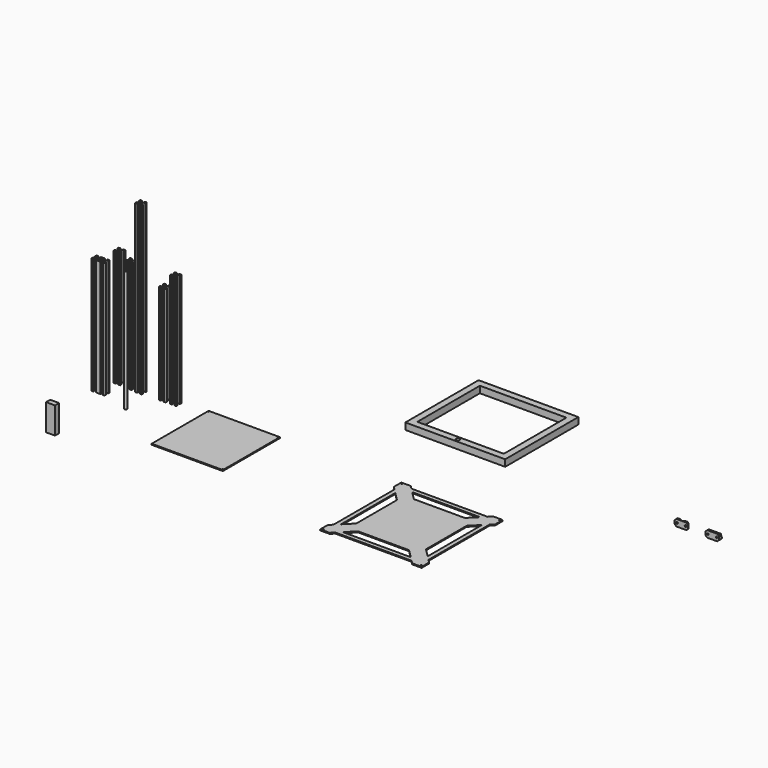
from build123d import *

# Parameters (mm, degrees)
F3_R         = 2.1
F4_DEPTH     = 350
F2_R         = 2.1
F5_DEPTH     = 500
F6_W         = 214
F6_H         = 214
F6_R         = 1.5
F7_DEPTH     = 3
F0_R         = 2.1
F8_DEPTH     = 350
F9_R         = 2
F10_DEPTH    = 3
F1_R         = 2.1
F11_DEPTH    = 335
F12_R        = 4
F13_DEPTH    = 365
F14_W        = 26.9409120083
F14_H        = 15.4066830873
F15_DEPTH    = 80
F16_R        = 2.1
F17_DEPTH    = 300
F18_R        = 2.1
F19_DEPTH    = 340
F20_R        = 5.6486540252
F20_W        = 260
F20_H        = 20
F21_DEPTH    = 20
F22_W        = 40
F22_H        = 15
F22_R        = 2
F23_DEPTH    = 20
F24_R        = 6
F25_DEPTH    = 10
F26_R        = 2.75
F27_DEPTH    = 25
F28_T1_DEPTH = 86.8637576871
F29_W        = 40
F29_H        = 23.6347752469
F29_R        = 2
F30_DEPTH    = 20
F31_R        = 6
F32_DEPTH    = 18
F33_R        = 2.25
F34_DEPTH    = 25
F35_T1_DEPTH = 81.7203917112
F36_W        = 47.229886055
F36_H        = 17.0893235207
F37_DEPTH    = 18
F38_SIZE     = 5
F39_W        = 52.9752969742
F39_H        = 17.0372793525
F40_DEPTH    = 10
F41_R        = 7.6141041327
F42_DEPTH    = 12
F43_SIZE     = 5
F44_SIZE     = 2


# Not quite as in the source:
# - a fillet or chamfer that OpenCascade refuses, or shapes differently, is made with other operations: its cross-section is extruded or revolved along the edge and cut away or added


with BuildPart() as f4:
    # F3 (on Top) → F4 (new body)
    with BuildSketch(Plane.XY):
        with BuildLine():
            Line((-71.2157925161, -12.9482020284), (-74.8085638019, -12.9482020284))
            ThreePointArc((-74.8085638019, -12.9482020284), (-75.8692239736, -13.3875418566), (-76.3085638019, -14.4482020284))
            Line((-76.3085638019, -14.4482020284), (-76.3085638019, -18.0409733141))
            ThreePointArc((-76.3085638019, -18.0409733141), (-76.2484286325, -18.3432932257), (-76.077178159, -18.5995876712))
            Line((-76.077178159, -18.5995876712), (-74.6185638019, -20.0582020284))
            Line((-74.6185638019, -20.0582020284), (-74.5085638019, -20.0582020284))
            Line((-74.5085638019, -20.0582020284), (-74.5085638019, -17.4482020284))
            Line((-74.5085638019, -17.4482020284), (-72.8692239736, -17.4482020284))
            Line((-72.8692239736, -17.4482020284), (-69.7085638019, -20.6088622002))
            Line((-69.7085638019, -20.6088622002), (-69.7085638019, -25.2875418566))
            Line((-69.7085638019, -25.2875418566), (-72.8692239736, -28.4482020284))
            Line((-72.8692239736, -28.4482020284), (-74.5085638019, -28.4482020284))
            Line((-74.5085638019, -28.4482020284), (-74.5085638019, -25.8382020284))
            Line((-74.5085638019, -25.8382020284), (-74.6185638019, -25.8382020284))
            Line((-74.6185638019, -25.8382020284), (-76.077178159, -27.2968163855))
            ThreePointArc((-76.077178159, -27.2968163855), (-76.2484286325, -27.5531108311), (-76.3085638019, -27.8554307427))
            Line((-76.3085638019, -27.8554307427), (-76.3085638019, -31.4482020284))
            ThreePointArc((-76.3085638019, -31.4482020284), (-75.8692239736, -32.5088622002), (-74.8085638019, -32.9482020284))
            Line((-74.8085638019, -32.9482020284), (-71.2157925161, -32.9482020284))
            ThreePointArc((-71.2157925161, -32.9482020284), (-70.9134726046, -32.8880668591), (-70.657178159, -32.7168163855))
            Line((-70.657178159, -32.7168163855), (-69.1985638019, -31.2582020284))
            Line((-69.1985638019, -31.2582020284), (-69.1985638019, -31.1482020284))
            Line((-69.1985638019, -31.1482020284), (-71.8085638019, -31.1482020284))
            Line((-71.8085638019, -31.1482020284), (-71.8085638019, -29.5088622002))
            Line((-71.8085638019, -29.5088622002), (-68.6479036301, -26.3482020284))
            Line((-68.6479036301, -26.3482020284), (-63.9692239736, -26.3482020284))
            Line((-63.9692239736, -26.3482020284), (-60.8085638019, -29.5088622002))
            Line((-60.8085638019, -29.5088622002), (-60.8085638019, -31.1482020284))
            Line((-60.8085638019, -31.1482020284), (-63.4185638019, -31.1482020284))
            Line((-63.4185638019, -31.1482020284), (-63.4185638019, -31.2582020284))
            Line((-63.4185638019, -31.2582020284), (-61.9599494447, -32.7168163855))
            ThreePointArc((-61.9599494447, -32.7168163855), (-61.7036549992, -32.8880668591), (-61.4013350876, -32.9482020284))
            Line((-61.4013350876, -32.9482020284), (-57.8085638019, -32.9482020284))
            Line((-57.8085638019, -32.9482020284), (-54.8085638019, -32.9482020284))
            Line((-54.8085638019, -32.9482020284), (-51.2157925161, -32.9482020284))
            ThreePointArc((-51.2157925161, -32.9482020284), (-50.9134726046, -32.8880668591), (-50.657178159, -32.7168163855))
            Line((-50.657178159, -32.7168163855), (-49.1985638019, -31.2582020284))
            Line((-49.1985638019, -31.2582020284), (-49.1985638019, -31.1482020284))
            Line((-49.1985638019, -31.1482020284), (-51.8085638019, -31.1482020284))
            Line((-51.8085638019, -31.1482020284), (-51.8085638019, -29.5088622002))
            Line((-51.8085638019, -29.5088622002), (-48.6479036301, -26.3482020284))
            Line((-48.6479036301, -26.3482020284), (-43.9692239736, -26.3482020284))
            Line((-43.9692239736, -26.3482020284), (-40.8085638019, -29.5088622002))
            Line((-40.8085638019, -29.5088622002), (-40.8085638019, -31.1482020284))
            Line((-40.8085638019, -31.1482020284), (-43.4185638019, -31.1482020284))
            Line((-43.4185638019, -31.1482020284), (-43.4185638019, -31.2582020284))
            Line((-43.4185638019, -31.2582020284), (-41.9599494447, -32.7168163855))
            ThreePointArc((-41.9599494447, -32.7168163855), (-41.7036549992, -32.8880668591), (-41.4013350876, -32.9482020284))
            Line((-41.4013350876, -32.9482020284), (-37.8085638019, -32.9482020284))
            ThreePointArc((-37.8085638019, -32.9482020284), (-36.7479036301, -32.5088622002), (-36.3085638019, -31.4482020284))
            Line((-36.3085638019, -31.4482020284), (-36.3085638019, -27.8554307427))
            ThreePointArc((-36.3085638019, -27.8554307427), (-36.3686989712, -27.5531108311), (-36.5399494447, -27.2968163855))
            Line((-36.5399494447, -27.2968163855), (-37.9985638019, -25.8382020284))
            Line((-37.9985638019, -25.8382020284), (-38.1085638019, -25.8382020284))
            Line((-38.1085638019, -25.8382020284), (-38.1085638019, -28.4482020284))
            Line((-38.1085638019, -28.4482020284), (-39.7479036301, -28.4482020284))
            Line((-39.7479036301, -28.4482020284), (-42.9085638019, -25.2875418566))
            Line((-42.9085638019, -25.2875418566), (-42.9085638019, -20.6088622002))
            Line((-42.9085638019, -20.6088622002), (-39.7479036301, -17.4482020284))
            Line((-39.7479036301, -17.4482020284), (-38.1085638019, -17.4482020284))
            Line((-38.1085638019, -17.4482020284), (-38.1085638019, -20.0582020284))
            Line((-38.1085638019, -20.0582020284), (-37.9985638019, -20.0582020284))
            Line((-37.9985638019, -20.0582020284), (-36.5399494447, -18.5995876712))
            ThreePointArc((-36.5399494447, -18.5995876712), (-36.3686989712, -18.3432932257), (-36.3085638019, -18.0409733141))
            Line((-36.3085638019, -18.0409733141), (-36.3085638019, -14.4482020284))
            ThreePointArc((-36.3085638019, -14.4482020284), (-36.7479036301, -13.3875418566), (-37.8085638019, -12.9482020284))
            Line((-37.8085638019, -12.9482020284), (-41.4013350876, -12.9482020284))
            ThreePointArc((-41.4013350876, -12.9482020284), (-41.7036549992, -13.0083371977), (-41.9599494447, -13.1795876712))
            Line((-41.9599494447, -13.1795876712), (-43.4185638019, -14.6382020284))
            Line((-43.4185638019, -14.6382020284), (-43.4185638019, -14.7482020284))
            Line((-43.4185638019, -14.7482020284), (-40.8085638019, -14.7482020284))
            Line((-40.8085638019, -14.7482020284), (-40.8085638019, -16.3875418566))
            Line((-40.8085638019, -16.3875418566), (-43.9692239736, -19.5482020284))
            Line((-43.9692239736, -19.5482020284), (-48.6479036301, -19.5482020284))
            Line((-48.6479036301, -19.5482020284), (-51.8085638019, -16.3875418566))
            Line((-51.8085638019, -16.3875418566), (-51.8085638019, -14.7482020284))
            Line((-51.8085638019, -14.7482020284), (-49.1985638019, -14.7482020284))
            Line((-49.1985638019, -14.7482020284), (-49.1985638019, -14.6382020284))
            Line((-49.1985638019, -14.6382020284), (-50.657178159, -13.1795876712))
            ThreePointArc((-50.657178159, -13.1795876712), (-50.9134726046, -13.0083371977), (-51.2157925161, -12.9482020284))
            Line((-51.2157925161, -12.9482020284), (-54.8085638019, -12.9482020284))
            Line((-54.8085638019, -12.9482020284), (-57.8085638019, -12.9482020284))
            Line((-57.8085638019, -12.9482020284), (-61.4013350876, -12.9482020284))
            ThreePointArc((-61.4013350876, -12.9482020284), (-61.7036549992, -13.0083371977), (-61.9599494447, -13.1795876712))
            Line((-61.9599494447, -13.1795876712), (-63.4185638019, -14.6382020284))
            Line((-63.4185638019, -14.6382020284), (-63.4185638019, -14.7482020284))
            Line((-63.4185638019, -14.7482020284), (-60.8085638019, -14.7482020284))
            Line((-60.8085638019, -14.7482020284), (-60.8085638019, -16.3875418566))
            Line((-60.8085638019, -16.3875418566), (-63.9692239736, -19.5482020284))
            Line((-63.9692239736, -19.5482020284), (-68.6479036301, -19.5482020284))
            Line((-68.6479036301, -19.5482020284), (-71.8085638019, -16.3875418566))
            Line((-71.8085638019, -16.3875418566), (-71.8085638019, -14.7482020284))
            Line((-71.8085638019, -14.7482020284), (-69.1985638019, -14.7482020284))
            Line((-69.1985638019, -14.7482020284), (-69.1985638019, -14.6382020284))
            Line((-69.1985638019, -14.6382020284), (-70.657178159, -13.1795876712))
            ThreePointArc((-70.657178159, -13.1795876712), (-70.9134726046, -13.0083371977), (-71.2157925161, -12.9482020284))
        make_face()
        Polygon((-74.5085638019, -29.5182020284), (-73.9685638019, -29.5182020284), (-72.8785638019, -30.6082020284), (-72.8785638019, -31.1482020284), (-74.5085638019, -31.1482020284), align=None, mode=Mode.SUBTRACT)
        Polygon((-58.6485638019, -29.5182020284), (-58.1085638019, -29.5182020284), (-58.1085638019, -31.1482020284), (-59.7385638019, -31.1482020284), (-59.7385638019, -30.6082020284), align=None, mode=Mode.SUBTRACT)
        Polygon((-54.5085638019, -31.1482020284), (-54.5085638019, -29.5182020284), (-53.9685638019, -29.5182020284), (-52.8785638019, -30.6082020284), (-52.8785638019, -31.1482020284), align=None, mode=Mode.SUBTRACT)
        Polygon((-39.7385638019, -30.6082020284), (-38.6485638019, -29.5182020284), (-38.1085638019, -29.5182020284), (-38.1085638019, -31.1482020284), (-39.7385638019, -31.1482020284), align=None, mode=Mode.SUBTRACT)
        with BuildLine():
            Line((-59.7479036301, -28.4482020284), (-62.9085638019, -25.2875418566))
            Line((-62.9085638019, -25.2875418566), (-62.9085638019, -23.6909259111))
            Line((-62.9085638019, -23.6909259111), (-58.2713541983, -23.6909259111))
            ThreePointArc((-58.2713541983, -23.6909259111), (-56.3085638019, -25.0468170256), (-54.3457734054, -23.6909259111))
            Line((-54.3457734054, -23.6909259111), (-49.7085638019, -23.6909259111))
            Line((-49.7085638019, -23.6909259111), (-49.7085638019, -25.2875418566))
            Line((-49.7085638019, -25.2875418566), (-52.8692239736, -28.4482020284))
            Line((-52.8692239736, -28.4482020284), (-54.5085638019, -28.4482020284))
            Line((-54.5085638019, -28.4482020284), (-58.1085638019, -28.4482020284))
            Line((-58.1085638019, -28.4482020284), (-59.7479036301, -28.4482020284))
        make_face(mode=Mode.SUBTRACT)
        with Locations((-66.3085638019, -22.9482020284)):
            Circle(F3_R, mode=Mode.SUBTRACT)
        Polygon((-74.5085638019, -14.7482020284), (-72.8785638019, -14.7482020284), (-72.8785638019, -15.2882020284), (-73.9685638019, -16.3782020284), (-74.5085638019, -16.3782020284), align=None, mode=Mode.SUBTRACT)
        Polygon((-58.1085638019, -14.7482020284), (-58.1085638019, -16.3782020284), (-58.6485638019, -16.3782020284), (-59.7385638019, -15.2882020284), (-59.7385638019, -14.7482020284), align=None, mode=Mode.SUBTRACT)
        with BuildLine():
            Line((-62.9085638019, -22.2054781457), (-62.9085638019, -20.6088622002))
            Line((-62.9085638019, -20.6088622002), (-59.7479036301, -17.4482020284))
            Line((-59.7479036301, -17.4482020284), (-58.1085638019, -17.4482020284))
            Line((-58.1085638019, -17.4482020284), (-54.5085638019, -17.4482020284))
            Line((-54.5085638019, -17.4482020284), (-52.8692239736, -17.4482020284))
            Line((-52.8692239736, -17.4482020284), (-49.7085638019, -20.6088622002))
            Line((-49.7085638019, -20.6088622002), (-49.7085638019, -22.2054781457))
            Line((-49.7085638019, -22.2054781457), (-54.3457734054, -22.2054781457))
            ThreePointArc((-54.3457734054, -22.2054781457), (-56.3085638019, -20.8495870312), (-58.2713541983, -22.2054781457))
            Line((-58.2713541983, -22.2054781457), (-62.9085638019, -22.2054781457))
        make_face(mode=Mode.SUBTRACT)
        with Locations((-46.3085638019, -22.9482020284)):
            Circle(F3_R, mode=Mode.SUBTRACT)
        Polygon((-52.8785638019, -15.2882020284), (-53.9685638019, -16.3782020284), (-54.5085638019, -16.3782020284), (-54.5085638019, -14.7482020284), (-52.8785638019, -14.7482020284), align=None, mode=Mode.SUBTRACT)
        Polygon((-38.6485638019, -16.3782020284), (-39.7385638019, -15.2882020284), (-39.7385638019, -14.7482020284), (-38.1085638019, -14.7482020284), (-38.1085638019, -16.3782020284), align=None, mode=Mode.SUBTRACT)
    extrude(amount=F4_DEPTH)


with BuildPart() as f5:
    # F2 (on Top) → F5 (new body)
    with BuildSketch(Plane.XY):
        with BuildLine():
            Line((12.9063250926, 46.0312701171), (9.3135538069, 46.0312701171))
            ThreePointArc((9.3135538069, 46.0312701171), (8.2528936351, 45.5919302888), (7.8135538069, 44.5312701171))
            Line((7.8135538069, 44.5312701171), (7.8135538069, 40.9384988313))
            ThreePointArc((7.8135538069, 40.9384988313), (7.8736889762, 40.6361789198), (8.0449394498, 40.3798844742))
            Line((8.0449394498, 40.3798844742), (9.5035538069, 38.9212701171))
            Line((9.5035538069, 38.9212701171), (9.6135538069, 38.9212701171))
            Line((9.6135538069, 38.9212701171), (9.6135538069, 41.5312701171))
            Line((9.6135538069, 41.5312701171), (11.2528936351, 41.5312701171))
            Line((11.2528936351, 41.5312701171), (14.4135538069, 38.3706099453))
            Line((14.4135538069, 38.3706099453), (14.4135538069, 33.6919302888))
            Line((14.4135538069, 33.6919302888), (11.2528936351, 30.5312701171))
            Line((11.2528936351, 30.5312701171), (9.6135538069, 30.5312701171))
            Line((9.6135538069, 30.5312701171), (9.6135538069, 33.1412701171))
            Line((9.6135538069, 33.1412701171), (9.5035538069, 33.1412701171))
            Line((9.5035538069, 33.1412701171), (8.0449394498, 31.6826557599))
            ThreePointArc((8.0449394498, 31.6826557599), (7.8736889762, 31.4263613144), (7.8135538069, 31.1240414028))
            Line((7.8135538069, 31.1240414028), (7.8135538069, 27.5312701171))
            ThreePointArc((7.8135538069, 27.5312701171), (8.2528936351, 26.4706099453), (9.3135538069, 26.0312701171))
            Line((9.3135538069, 26.0312701171), (12.9063250926, 26.0312701171))
            ThreePointArc((12.9063250926, 26.0312701171), (13.2086450042, 26.0914052864), (13.4649394498, 26.2626557599))
            Line((13.4649394498, 26.2626557599), (14.9235538069, 27.7212701171))
            Line((14.9235538069, 27.7212701171), (14.9235538069, 27.8312701171))
            Line((14.9235538069, 27.8312701171), (12.3135538069, 27.8312701171))
            Line((12.3135538069, 27.8312701171), (12.3135538069, 29.4706099453))
            Line((12.3135538069, 29.4706099453), (15.4742139787, 32.6312701171))
            Line((15.4742139787, 32.6312701171), (20.1528936351, 32.6312701171))
            Line((20.1528936351, 32.6312701171), (23.3135538069, 29.4706099453))
            Line((23.3135538069, 29.4706099453), (23.3135538069, 27.8312701171))
            Line((23.3135538069, 27.8312701171), (20.7035538069, 27.8312701171))
            Line((20.7035538069, 27.8312701171), (20.7035538069, 27.7212701171))
            Line((20.7035538069, 27.7212701171), (22.1621681641, 26.2626557599))
            ThreePointArc((22.1621681641, 26.2626557599), (22.4184626096, 26.0914052864), (22.7207825212, 26.0312701171))
            Line((22.7207825212, 26.0312701171), (26.3135538069, 26.0312701171))
            ThreePointArc((26.3135538069, 26.0312701171), (27.3742139787, 26.4706099453), (27.8135538069, 27.5312701171))
            Line((27.8135538069, 27.5312701171), (27.8135538069, 31.1240414028))
            ThreePointArc((27.8135538069, 31.1240414028), (27.7534186376, 31.4263613144), (27.5821681641, 31.6826557599))
            Line((27.5821681641, 31.6826557599), (26.1235538069, 33.1412701171))
            Line((26.1235538069, 33.1412701171), (26.0135538069, 33.1412701171))
            Line((26.0135538069, 33.1412701171), (26.0135538069, 30.5312701171))
            Line((26.0135538069, 30.5312701171), (24.3742139787, 30.5312701171))
            Line((24.3742139787, 30.5312701171), (21.2135538069, 33.6919302888))
            Line((21.2135538069, 33.6919302888), (21.2135538069, 38.3706099453))
            Line((21.2135538069, 38.3706099453), (24.3742139787, 41.5312701171))
            Line((24.3742139787, 41.5312701171), (26.0135538069, 41.5312701171))
            Line((26.0135538069, 41.5312701171), (26.0135538069, 38.9212701171))
            Line((26.0135538069, 38.9212701171), (26.1235538069, 38.9212701171))
            Line((26.1235538069, 38.9212701171), (27.5821681641, 40.3798844742))
            ThreePointArc((27.5821681641, 40.3798844742), (27.7534186376, 40.6361789198), (27.8135538069, 40.9384988313))
            Line((27.8135538069, 40.9384988313), (27.8135538069, 44.5312701171))
            ThreePointArc((27.8135538069, 44.5312701171), (27.3742139787, 45.5919302888), (26.3135538069, 46.0312701171))
            Line((26.3135538069, 46.0312701171), (22.7207825212, 46.0312701171))
            ThreePointArc((22.7207825212, 46.0312701171), (22.4184626096, 45.9711349477), (22.1621681641, 45.7998844742))
            Line((22.1621681641, 45.7998844742), (20.7035538069, 44.3412701171))
            Line((20.7035538069, 44.3412701171), (20.7035538069, 44.2312701171))
            Line((20.7035538069, 44.2312701171), (23.3135538069, 44.2312701171))
            Line((23.3135538069, 44.2312701171), (23.3135538069, 42.5919302888))
            Line((23.3135538069, 42.5919302888), (20.1528936351, 39.4312701171))
            Line((20.1528936351, 39.4312701171), (15.4742139787, 39.4312701171))
            Line((15.4742139787, 39.4312701171), (12.3135538069, 42.5919302888))
            Line((12.3135538069, 42.5919302888), (12.3135538069, 44.2312701171))
            Line((12.3135538069, 44.2312701171), (14.9235538069, 44.2312701171))
            Line((14.9235538069, 44.2312701171), (14.9235538069, 44.3412701171))
            Line((14.9235538069, 44.3412701171), (13.4649394498, 45.7998844742))
            ThreePointArc((13.4649394498, 45.7998844742), (13.2086450042, 45.9711349477), (12.9063250926, 46.0312701171))
        make_face()
        Polygon((9.6135538069, 29.4612701171), (10.1535538069, 29.4612701171), (11.2435538069, 28.3712701171), (11.2435538069, 27.8312701171), (9.6135538069, 27.8312701171), align=None, mode=Mode.SUBTRACT)
        Polygon((25.4735538069, 29.4612701171), (26.0135538069, 29.4612701171), (26.0135538069, 27.8312701171), (24.3835538069, 27.8312701171), (24.3835538069, 28.3712701171), align=None, mode=Mode.SUBTRACT)
        with Locations((17.8135538069, 36.0312701171)):
            Circle(F2_R, mode=Mode.SUBTRACT)
        Polygon((9.6135538069, 44.2312701171), (11.2435538069, 44.2312701171), (11.2435538069, 43.6912701171), (10.1535538069, 42.6012701171), (9.6135538069, 42.6012701171), align=None, mode=Mode.SUBTRACT)
        Polygon((26.0135538069, 44.2312701171), (26.0135538069, 42.6012701171), (25.4735538069, 42.6012701171), (24.3835538069, 43.6912701171), (24.3835538069, 44.2312701171), align=None, mode=Mode.SUBTRACT)
    extrude(amount=F5_DEPTH)


with BuildPart() as f7:
    # F6 (on Top) → F7 (new body)
    with BuildSketch(Plane.XY):
        with Locations((313.2716193795, -52.2007276407)):
            Rectangle(F6_W, F6_H)
        with Locations((208.7716193795, -156.7007276407)):
            Circle(F6_R, mode=Mode.SUBTRACT)
        with Locations((417.7716193795, -156.7007276407)):
            Circle(F6_R, mode=Mode.SUBTRACT)
        with Locations((208.7716193795, 52.2992723593)):
            Circle(F6_R, mode=Mode.SUBTRACT)
        with Locations((417.7716193795, 52.2992723593)):
            Circle(F6_R, mode=Mode.SUBTRACT)
    extrude(amount=F7_DEPTH)


with BuildPart() as f8:
    # F0 (on Top) → F8 (new body)
    with BuildSketch(Plane.XY):
        with BuildLine():
            Line((-55.2372885438, 50.4958480005), (-58.8300598296, 50.4958480005))
            ThreePointArc((-58.8300598296, 50.4958480005), (-59.8907200014, 50.0565081723), (-60.3300598296, 48.9958480005))
            Line((-60.3300598296, 48.9958480005), (-60.3300598296, 45.4030767148))
            ThreePointArc((-60.3300598296, 45.4030767148), (-60.2699246603, 45.1007568032), (-60.0986741867, 44.8444623577))
            Line((-60.0986741867, 44.8444623577), (-58.6400598296, 43.3858480005))
            Line((-58.6400598296, 43.3858480005), (-58.5300598296, 43.3858480005))
            Line((-58.5300598296, 43.3858480005), (-58.5300598296, 45.9958480005))
            Line((-58.5300598296, 45.9958480005), (-56.8907200014, 45.9958480005))
            Line((-56.8907200014, 45.9958480005), (-53.7300598296, 42.8351878288))
            Line((-53.7300598296, 42.8351878288), (-53.7300598296, 38.1565081723))
            Line((-53.7300598296, 38.1565081723), (-56.8907200014, 34.9958480005))
            Line((-56.8907200014, 34.9958480005), (-58.5300598296, 34.9958480005))
            Line((-58.5300598296, 34.9958480005), (-58.5300598296, 37.6058480005))
            Line((-58.5300598296, 37.6058480005), (-58.6400598296, 37.6058480005))
            Line((-58.6400598296, 37.6058480005), (-60.0986741867, 36.1472336434))
            ThreePointArc((-60.0986741867, 36.1472336434), (-60.2699246603, 35.8909391978), (-60.3300598296, 35.5886192863))
            Line((-60.3300598296, 35.5886192863), (-60.3300598296, 31.9958480005))
            ThreePointArc((-60.3300598296, 31.9958480005), (-59.8907200014, 30.9351878288), (-58.8300598296, 30.4958480005))
            Line((-58.8300598296, 30.4958480005), (-55.2372885438, 30.4958480005))
            ThreePointArc((-55.2372885438, 30.4958480005), (-54.9349686323, 30.5559831699), (-54.6786741867, 30.7272336434))
            Line((-54.6786741867, 30.7272336434), (-53.2200598296, 32.1858480005))
            Line((-53.2200598296, 32.1858480005), (-53.2200598296, 32.2958480005))
            Line((-53.2200598296, 32.2958480005), (-55.8300598296, 32.2958480005))
            Line((-55.8300598296, 32.2958480005), (-55.8300598296, 33.9351878288))
            Line((-55.8300598296, 33.9351878288), (-52.6693996578, 37.0958480005))
            Line((-52.6693996578, 37.0958480005), (-47.9907200014, 37.0958480005))
            Line((-47.9907200014, 37.0958480005), (-44.8300598296, 33.9351878288))
            Line((-44.8300598296, 33.9351878288), (-44.8300598296, 32.2958480005))
            Line((-44.8300598296, 32.2958480005), (-47.4400598296, 32.2958480005))
            Line((-47.4400598296, 32.2958480005), (-47.4400598296, 32.1858480005))
            Line((-47.4400598296, 32.1858480005), (-45.9814454724, 30.7272336434))
            ThreePointArc((-45.9814454724, 30.7272336434), (-45.7251510269, 30.5559831699), (-45.4228311153, 30.4958480005))
            Line((-45.4228311153, 30.4958480005), (-41.8300598296, 30.4958480005))
            ThreePointArc((-41.8300598296, 30.4958480005), (-40.7693996578, 30.9351878288), (-40.3300598296, 31.9958480005))
            Line((-40.3300598296, 31.9958480005), (-40.3300598296, 35.5886192863))
            ThreePointArc((-40.3300598296, 35.5886192863), (-40.3901949989, 35.8909391978), (-40.5614454724, 36.1472336434))
            Line((-40.5614454724, 36.1472336434), (-42.0200598296, 37.6058480005))
            Line((-42.0200598296, 37.6058480005), (-42.1300598296, 37.6058480005))
            Line((-42.1300598296, 37.6058480005), (-42.1300598296, 34.9958480005))
            Line((-42.1300598296, 34.9958480005), (-43.7693996578, 34.9958480005))
            Line((-43.7693996578, 34.9958480005), (-46.9300598296, 38.1565081723))
            Line((-46.9300598296, 38.1565081723), (-46.9300598296, 42.8351878288))
            Line((-46.9300598296, 42.8351878288), (-43.7693996578, 45.9958480005))
            Line((-43.7693996578, 45.9958480005), (-42.1300598296, 45.9958480005))
            Line((-42.1300598296, 45.9958480005), (-42.1300598296, 43.3858480005))
            Line((-42.1300598296, 43.3858480005), (-42.0200598296, 43.3858480005))
            Line((-42.0200598296, 43.3858480005), (-40.5614454724, 44.8444623577))
            ThreePointArc((-40.5614454724, 44.8444623577), (-40.3901949989, 45.1007568032), (-40.3300598296, 45.4030767148))
            Line((-40.3300598296, 45.4030767148), (-40.3300598296, 48.9958480005))
            ThreePointArc((-40.3300598296, 48.9958480005), (-40.7693996578, 50.0565081723), (-41.8300598296, 50.4958480005))
            Line((-41.8300598296, 50.4958480005), (-45.4228311153, 50.4958480005))
            ThreePointArc((-45.4228311153, 50.4958480005), (-45.7251510269, 50.4357128312), (-45.9814454724, 50.2644623577))
            Line((-45.9814454724, 50.2644623577), (-47.4400598296, 48.8058480005))
            Line((-47.4400598296, 48.8058480005), (-47.4400598296, 48.6958480005))
            Line((-47.4400598296, 48.6958480005), (-44.8300598296, 48.6958480005))
            Line((-44.8300598296, 48.6958480005), (-44.8300598296, 47.0565081723))
            Line((-44.8300598296, 47.0565081723), (-47.9907200014, 43.8958480005))
            Line((-47.9907200014, 43.8958480005), (-52.6693996578, 43.8958480005))
            Line((-52.6693996578, 43.8958480005), (-55.8300598296, 47.0565081723))
            Line((-55.8300598296, 47.0565081723), (-55.8300598296, 48.6958480005))
            Line((-55.8300598296, 48.6958480005), (-53.2200598296, 48.6958480005))
            Line((-53.2200598296, 48.6958480005), (-53.2200598296, 48.8058480005))
            Line((-53.2200598296, 48.8058480005), (-54.6786741867, 50.2644623577))
            ThreePointArc((-54.6786741867, 50.2644623577), (-54.9349686323, 50.4357128312), (-55.2372885438, 50.4958480005))
        make_face()
        Polygon((-58.5300598296, 33.9258480005), (-57.9900598296, 33.9258480005), (-56.9000598296, 32.8358480005), (-56.9000598296, 32.2958480005), (-58.5300598296, 32.2958480005), align=None, mode=Mode.SUBTRACT)
        Polygon((-42.6700598296, 33.9258480005), (-42.1300598296, 33.9258480005), (-42.1300598296, 32.2958480005), (-43.7600598296, 32.2958480005), (-43.7600598296, 32.8358480005), align=None, mode=Mode.SUBTRACT)
        with Locations((-50.3300598296, 40.4958480005)):
            Circle(F0_R, mode=Mode.SUBTRACT)
        Polygon((-58.5300598296, 48.6958480005), (-56.9000598296, 48.6958480005), (-56.9000598296, 48.1558480005), (-57.9900598296, 47.0658480005), (-58.5300598296, 47.0658480005), align=None, mode=Mode.SUBTRACT)
        Polygon((-42.1300598296, 48.6958480005), (-42.1300598296, 47.0658480005), (-42.6700598296, 47.0658480005), (-43.7600598296, 48.1558480005), (-43.7600598296, 48.6958480005), align=None, mode=Mode.SUBTRACT)
        with BuildLine():
            ThreePointArc((-60.3300598296, 48.9958480005), (-59.8907200014, 50.0565081723), (-58.8300598296, 50.4958480005))
            Line((-58.8300598296, 50.4958480005), (-60.3300598296, 50.4958480005))
            Line((-60.3300598296, 50.4958480005), (-60.3300598296, 48.9958480005))
        make_face()
        with BuildLine():
            Line((-40.3300598296, 50.4958480005), (-41.8300598296, 50.4958480005))
            ThreePointArc((-41.8300598296, 50.4958480005), (-40.7693996578, 50.0565081723), (-40.3300598296, 48.9958480005))
            Line((-40.3300598296, 48.9958480005), (-40.3300598296, 50.4958480005))
        make_face()
        with BuildLine():
            ThreePointArc((-58.8300598296, 30.4958480005), (-59.8907200014, 30.9351878288), (-60.3300598296, 31.9958480005))
            Line((-60.3300598296, 31.9958480005), (-60.3300598296, 30.4958480005))
            Line((-60.3300598296, 30.4958480005), (-58.8300598296, 30.4958480005))
        make_face()
        with BuildLine():
            Line((-40.3300598296, 30.4958480005), (-40.3300598296, 31.9958480005))
            ThreePointArc((-40.3300598296, 31.9958480005), (-40.7693996578, 30.9351878288), (-41.8300598296, 30.4958480005))
            Line((-41.8300598296, 30.4958480005), (-40.3300598296, 30.4958480005))
        make_face()
    extrude(amount=F8_DEPTH)


with BuildPart() as f10:
    # F9 (on Top) → F10 (new body)
    with BuildSketch(Plane.XY):
        with BuildLine():
            Line((815.4132323337, 52.85364175), (792.1289610863, 52.85364175))
            ThreePointArc((792.1289610863, 52.85364175), (788.5934271803, 51.3891756559), (787.1289610863, 47.85364175))
            Line((787.1289610863, 47.85364175), (787.1289610863, 24.5693705025))
            Line((787.1289610863, 24.5693705025), (796.6539610863, 15.0443705025))
            Line((796.6539610863, 15.0443705025), (796.6539610863, 43.32864175))
            Line((796.6539610863, 43.32864175), (824.9382323337, 43.32864175))
            Line((824.9382323337, 43.32864175), (815.4132323337, 52.85364175))
        make_face()
        with Locations((791.8914610863, 48.09114175)):
            Circle(F9_R, mode=Mode.SUBTRACT)
        with BuildLine():
            ThreePointArc((787.1289610863, 47.85364175), (788.5934271803, 51.3891756559), (792.1289610863, 52.85364175))
            Line((792.1289610863, 52.85364175), (787.1289610863, 52.85364175))
            Line((787.1289610863, 52.85364175), (787.1289610863, 47.85364175))
        make_face()
        Polygon((1054.1196898388, 43.32864175), (824.9382323337, 43.32864175), (796.6539610863, 43.32864175), (796.6539610863, 15.0443705025), (796.6539610863, -214.1370870026), (796.6539610863, -242.42135825), (824.9382323337, -242.42135825), (1054.1196898388, -242.42135825), (1082.4039610863, -242.42135825), (1082.4039610863, -214.1370870026), (1082.4039610863, 15.0443705025), (1082.4039610863, 43.32864175), align=None)
        Polygon((863.0382323337, -204.32135825), (1016.0196898388, -204.32135825), (1041.4196898388, -229.72135825), (931.5041899681, -229.72135825), (837.6382323337, -229.72135825), align=None, mode=Mode.SUBTRACT)
        Polygon((834.7539610863, -23.0556294975), (834.7539610863, -176.0370870026), (809.3539610863, -201.4370870026), (809.3539610863, -104.5096218586), (809.3539610863, 2.3443705025), align=None, mode=Mode.SUBTRACT)
        Polygon((1041.4196898388, 30.62864175), (1016.0196898388, 5.22864175), (863.0382323337, 5.22864175), (837.6382323337, 30.62864175), (931.5041899681, 30.62864175), align=None, mode=Mode.SUBTRACT)
        Polygon((1069.7039610863, -201.4370870026), (1044.3039610863, -176.0370870026), (1044.3039610863, -23.0556294975), (1069.7039610863, 2.3443705025), (1069.7039610863, -104.5096218586), align=None, mode=Mode.SUBTRACT)
        with BuildLine():
            Line((1063.6446898388, 52.85364175), (1054.1196898388, 43.32864175))
            Line((1054.1196898388, 43.32864175), (1082.4039610863, 43.32864175))
            Line((1082.4039610863, 43.32864175), (1082.4039610863, 15.0443705025))
            Line((1082.4039610863, 15.0443705025), (1091.9289610863, 24.5693705025))
            Line((1091.9289610863, 24.5693705025), (1091.9289610863, 47.85364175))
            ThreePointArc((1091.9289610863, 47.85364175), (1090.4644949922, 51.3891756559), (1086.9289610863, 52.85364175))
            Line((1086.9289610863, 52.85364175), (1063.6446898388, 52.85364175))
        make_face()
        with Locations((1087.1664610863, 48.09114175)):
            Circle(F9_R, mode=Mode.SUBTRACT)
        with BuildLine():
            Line((796.6539610863, -242.42135825), (796.6539610863, -214.1370870026))
            Line((796.6539610863, -214.1370870026), (787.1289610863, -223.6620870026))
            Line((787.1289610863, -223.6620870026), (787.1289610863, -246.94635825))
            ThreePointArc((787.1289610863, -246.94635825), (788.5934271803, -250.481892156), (792.1289610863, -251.94635825))
            Line((792.1289610863, -251.94635825), (815.4132323337, -251.94635825))
            Line((815.4132323337, -251.94635825), (824.9382323337, -242.42135825))
            Line((824.9382323337, -242.42135825), (796.6539610863, -242.42135825))
        make_face()
        with Locations((791.8914610863, -247.18385825)):
            Circle(F9_R, mode=Mode.SUBTRACT)
        with BuildLine():
            Line((1091.9289610863, 52.85364175), (1086.9289610863, 52.85364175))
            ThreePointArc((1086.9289610863, 52.85364175), (1090.4644949922, 51.3891756559), (1091.9289610863, 47.85364175))
            Line((1091.9289610863, 47.85364175), (1091.9289610863, 52.85364175))
        make_face()
        with BuildLine():
            Line((1091.9289610863, -223.6620870026), (1082.4039610863, -214.1370870026))
            Line((1082.4039610863, -214.1370870026), (1082.4039610863, -242.42135825))
            Line((1082.4039610863, -242.42135825), (1054.1196898388, -242.42135825))
            Line((1054.1196898388, -242.42135825), (1063.6446898388, -251.94635825))
            Line((1063.6446898388, -251.94635825), (1086.9289610863, -251.94635825))
            ThreePointArc((1086.9289610863, -251.94635825), (1090.4644949922, -250.481892156), (1091.9289610863, -246.94635825))
            Line((1091.9289610863, -246.94635825), (1091.9289610863, -223.6620870026))
        make_face()
        with Locations((1087.1664610863, -247.18385825)):
            Circle(F9_R, mode=Mode.SUBTRACT)
        with BuildLine():
            ThreePointArc((792.1289610863, -251.94635825), (788.5934271803, -250.481892156), (787.1289610863, -246.94635825))
            Line((787.1289610863, -246.94635825), (787.1289610863, -251.94635825))
            Line((787.1289610863, -251.94635825), (792.1289610863, -251.94635825))
        make_face()
        with BuildLine():
            Line((1091.9289610863, -251.94635825), (1091.9289610863, -246.94635825))
            ThreePointArc((1091.9289610863, -246.94635825), (1090.4644949922, -250.481892156), (1086.9289610863, -251.94635825))
            Line((1086.9289610863, -251.94635825), (1091.9289610863, -251.94635825))
        make_face()
    extrude(amount=F10_DEPTH)


with BuildPart() as f11:
    # F1 (on Top) → F11 (new body)
    with BuildSketch(Plane.XY):
        with BuildLine():
            Line((-19.520636605, 48.3810491269), (-23.1134078907, 48.3810491269))
            ThreePointArc((-23.1134078907, 48.3810491269), (-24.1740680625, 47.9417092987), (-24.6134078907, 46.8810491269))
            Line((-24.6134078907, 46.8810491269), (-24.6134078907, 43.2882778412))
            ThreePointArc((-24.6134078907, 43.2882778412), (-24.5532727214, 42.9859579296), (-24.3820222479, 42.729663484))
            Line((-24.3820222479, 42.729663484), (-22.9234078907, 41.2710491269))
            Line((-22.9234078907, 41.2710491269), (-22.8134078907, 41.2710491269))
            Line((-22.8134078907, 41.2710491269), (-22.8134078907, 43.8810491269))
            Line((-22.8134078907, 43.8810491269), (-21.1740680625, 43.8810491269))
            Line((-21.1740680625, 43.8810491269), (-18.0134078907, 40.7203889551))
            Line((-18.0134078907, 40.7203889551), (-18.0134078907, 36.0417092987))
            Line((-18.0134078907, 36.0417092987), (-21.1740680625, 32.8810491269))
            Line((-21.1740680625, 32.8810491269), (-22.8134078907, 32.8810491269))
            Line((-22.8134078907, 32.8810491269), (-22.8134078907, 35.4910491269))
            Line((-22.8134078907, 35.4910491269), (-22.9234078907, 35.4910491269))
            Line((-22.9234078907, 35.4910491269), (-24.3820222479, 34.0324347697))
            ThreePointArc((-24.3820222479, 34.0324347697), (-24.5532727214, 33.7761403242), (-24.6134078907, 33.4738204126))
            Line((-24.6134078907, 33.4738204126), (-24.6134078907, 29.8810491269))
            ThreePointArc((-24.6134078907, 29.8810491269), (-24.1740680625, 28.8203889551), (-23.1134078907, 28.3810491269))
            Line((-23.1134078907, 28.3810491269), (-19.520636605, 28.3810491269))
            ThreePointArc((-19.520636605, 28.3810491269), (-19.2183166934, 28.4411842962), (-18.9620222479, 28.6124347697))
            Line((-18.9620222479, 28.6124347697), (-17.5034078907, 30.0710491269))
            Line((-17.5034078907, 30.0710491269), (-17.5034078907, 30.1810491269))
            Line((-17.5034078907, 30.1810491269), (-20.1134078907, 30.1810491269))
            Line((-20.1134078907, 30.1810491269), (-20.1134078907, 31.8203889551))
            Line((-20.1134078907, 31.8203889551), (-16.9527477189, 34.9810491269))
            Line((-16.9527477189, 34.9810491269), (-12.2740680625, 34.9810491269))
            Line((-12.2740680625, 34.9810491269), (-9.1134078907, 31.8203889551))
            Line((-9.1134078907, 31.8203889551), (-9.1134078907, 30.1810491269))
            Line((-9.1134078907, 30.1810491269), (-11.7234078907, 30.1810491269))
            Line((-11.7234078907, 30.1810491269), (-11.7234078907, 30.0710491269))
            Line((-11.7234078907, 30.0710491269), (-10.2647935336, 28.6124347697))
            ThreePointArc((-10.2647935336, 28.6124347697), (-10.008499088, 28.4411842962), (-9.7061791764, 28.3810491269))
            Line((-9.7061791764, 28.3810491269), (-6.1134078907, 28.3810491269))
            ThreePointArc((-6.1134078907, 28.3810491269), (-5.0527477189, 28.8203889551), (-4.6134078907, 29.8810491269))
            Line((-4.6134078907, 29.8810491269), (-4.6134078907, 33.4738204126))
            ThreePointArc((-4.6134078907, 33.4738204126), (-4.67354306, 33.7761403242), (-4.8447935336, 34.0324347697))
            Line((-4.8447935336, 34.0324347697), (-6.3034078907, 35.4910491269))
            Line((-6.3034078907, 35.4910491269), (-6.4134078907, 35.4910491269))
            Line((-6.4134078907, 35.4910491269), (-6.4134078907, 32.8810491269))
            Line((-6.4134078907, 32.8810491269), (-8.0527477189, 32.8810491269))
            Line((-8.0527477189, 32.8810491269), (-11.2134078907, 36.0417092987))
            Line((-11.2134078907, 36.0417092987), (-11.2134078907, 40.7203889551))
            Line((-11.2134078907, 40.7203889551), (-8.0527477189, 43.8810491269))
            Line((-8.0527477189, 43.8810491269), (-6.4134078907, 43.8810491269))
            Line((-6.4134078907, 43.8810491269), (-6.4134078907, 41.2710491269))
            Line((-6.4134078907, 41.2710491269), (-6.3034078907, 41.2710491269))
            Line((-6.3034078907, 41.2710491269), (-4.8447935336, 42.729663484))
            ThreePointArc((-4.8447935336, 42.729663484), (-4.67354306, 42.9859579296), (-4.6134078907, 43.2882778412))
            Line((-4.6134078907, 43.2882778412), (-4.6134078907, 46.8810491269))
            ThreePointArc((-4.6134078907, 46.8810491269), (-5.0527477189, 47.9417092987), (-6.1134078907, 48.3810491269))
            Line((-6.1134078907, 48.3810491269), (-9.7061791764, 48.3810491269))
            ThreePointArc((-9.7061791764, 48.3810491269), (-10.008499088, 48.3209139576), (-10.2647935336, 48.149663484))
            Line((-10.2647935336, 48.149663484), (-11.7234078907, 46.6910491269))
            Line((-11.7234078907, 46.6910491269), (-11.7234078907, 46.5810491269))
            Line((-11.7234078907, 46.5810491269), (-9.1134078907, 46.5810491269))
            Line((-9.1134078907, 46.5810491269), (-9.1134078907, 44.9417092987))
            Line((-9.1134078907, 44.9417092987), (-12.2740680625, 41.7810491269))
            Line((-12.2740680625, 41.7810491269), (-16.9527477189, 41.7810491269))
            Line((-16.9527477189, 41.7810491269), (-20.1134078907, 44.9417092987))
            Line((-20.1134078907, 44.9417092987), (-20.1134078907, 46.5810491269))
            Line((-20.1134078907, 46.5810491269), (-17.5034078907, 46.5810491269))
            Line((-17.5034078907, 46.5810491269), (-17.5034078907, 46.6910491269))
            Line((-17.5034078907, 46.6910491269), (-18.9620222479, 48.149663484))
            ThreePointArc((-18.9620222479, 48.149663484), (-19.2183166934, 48.3209139576), (-19.520636605, 48.3810491269))
        make_face()
        Polygon((-22.8134078907, 31.8110491269), (-22.2734078907, 31.8110491269), (-21.1834078907, 30.7210491269), (-21.1834078907, 30.1810491269), (-22.8134078907, 30.1810491269), align=None, mode=Mode.SUBTRACT)
        Polygon((-6.9534078907, 31.8110491269), (-6.4134078907, 31.8110491269), (-6.4134078907, 30.1810491269), (-8.0434078907, 30.1810491269), (-8.0434078907, 30.7210491269), align=None, mode=Mode.SUBTRACT)
        Polygon((-22.8134078907, 46.5810491269), (-21.1834078907, 46.5810491269), (-21.1834078907, 46.0410491269), (-22.2734078907, 44.9510491269), (-22.8134078907, 44.9510491269), align=None, mode=Mode.SUBTRACT)
        with Locations((-14.6134078907, 38.3810491269)):
            Circle(F1_R, mode=Mode.SUBTRACT)
        Polygon((-6.4134078907, 46.5810491269), (-6.4134078907, 44.9510491269), (-6.9534078907, 44.9510491269), (-8.0434078907, 46.0410491269), (-8.0434078907, 46.5810491269), align=None, mode=Mode.SUBTRACT)
    extrude(amount=F11_DEPTH)


with BuildPart() as f13:
    # F12 (on Top) → F13 (new body)
    with BuildSketch(Plane.XY):
        with Locations((43.8524484634, -54.1962496936)):
            Circle(F12_R)
    extrude(amount=F13_DEPTH)


with BuildPart() as f15:
    # F14 (on Top) → F15 (new body)
    with BuildSketch(Plane.XY):
        with Locations((-13.4704560041, -256.7725405097)):
            Rectangle(F14_W, F14_H)
    extrude(amount=F15_DEPTH)


with BuildPart() as f17:
    # F16 (on Top) → F17 (new body)
    with BuildSketch(Plane.XY):
        with BuildLine():
            Line((82.2794074622, 49.2925159042), (78.6866361765, 49.2925159042))
            ThreePointArc((78.6866361765, 49.2925159042), (77.6259760047, 48.853176076), (77.1866361765, 47.7925159042))
            Line((77.1866361765, 47.7925159042), (77.1866361765, 44.1997446185))
            ThreePointArc((77.1866361765, 44.1997446185), (77.2467713458, 43.8974247069), (77.4180218194, 43.6411302613))
            Line((77.4180218194, 43.6411302613), (78.8766361765, 42.1825159042))
            Line((78.8766361765, 42.1825159042), (78.9866361765, 42.1825159042))
            Line((78.9866361765, 42.1825159042), (78.9866361765, 44.7925159042))
            Line((78.9866361765, 44.7925159042), (80.6259760047, 44.7925159042))
            Line((80.6259760047, 44.7925159042), (83.7866361765, 41.6318557324))
            Line((83.7866361765, 41.6318557324), (83.7866361765, 36.953176076))
            Line((83.7866361765, 36.953176076), (80.6259760047, 33.7925159042))
            Line((80.6259760047, 33.7925159042), (78.9866361765, 33.7925159042))
            Line((78.9866361765, 33.7925159042), (78.9866361765, 36.4025159042))
            Line((78.9866361765, 36.4025159042), (78.8766361765, 36.4025159042))
            Line((78.8766361765, 36.4025159042), (77.4180218194, 34.9439015471))
            ThreePointArc((77.4180218194, 34.9439015471), (77.2467713458, 34.6876071015), (77.1866361765, 34.3852871899))
            Line((77.1866361765, 34.3852871899), (77.1866361765, 30.7925159042))
            ThreePointArc((77.1866361765, 30.7925159042), (77.6259760047, 29.7318557324), (78.6866361765, 29.2925159042))
            Line((78.6866361765, 29.2925159042), (82.2794074622, 29.2925159042))
            ThreePointArc((82.2794074622, 29.2925159042), (82.5817273738, 29.3526510735), (82.8380218194, 29.5239015471))
            Line((82.8380218194, 29.5239015471), (84.2966361765, 30.9825159042))
            Line((84.2966361765, 30.9825159042), (84.2966361765, 31.0925159042))
            Line((84.2966361765, 31.0925159042), (81.6866361765, 31.0925159042))
            Line((81.6866361765, 31.0925159042), (81.6866361765, 32.7318557324))
            Line((81.6866361765, 32.7318557324), (84.8472963483, 35.8925159042))
            Line((84.8472963483, 35.8925159042), (89.5259760047, 35.8925159042))
            Line((89.5259760047, 35.8925159042), (92.6866361765, 32.7318557324))
            Line((92.6866361765, 32.7318557324), (92.6866361765, 31.0925159042))
            Line((92.6866361765, 31.0925159042), (90.0766361765, 31.0925159042))
            Line((90.0766361765, 31.0925159042), (90.0766361765, 30.9825159042))
            Line((90.0766361765, 30.9825159042), (91.5352505336, 29.5239015471))
            ThreePointArc((91.5352505336, 29.5239015471), (91.7915449792, 29.3526510735), (92.0938648908, 29.2925159042))
            Line((92.0938648908, 29.2925159042), (95.6866361765, 29.2925159042))
            ThreePointArc((95.6866361765, 29.2925159042), (96.7472963483, 29.7318557324), (97.1866361765, 30.7925159042))
            Line((97.1866361765, 30.7925159042), (97.1866361765, 34.3852871899))
            ThreePointArc((97.1866361765, 34.3852871899), (97.1265010072, 34.6876071015), (96.9552505336, 34.9439015471))
            Line((96.9552505336, 34.9439015471), (95.4966361765, 36.4025159042))
            Line((95.4966361765, 36.4025159042), (95.3866361765, 36.4025159042))
            Line((95.3866361765, 36.4025159042), (95.3866361765, 33.7925159042))
            Line((95.3866361765, 33.7925159042), (93.7472963483, 33.7925159042))
            Line((93.7472963483, 33.7925159042), (90.5866361765, 36.953176076))
            Line((90.5866361765, 36.953176076), (90.5866361765, 41.6318557324))
            Line((90.5866361765, 41.6318557324), (93.7472963483, 44.7925159042))
            Line((93.7472963483, 44.7925159042), (95.3866361765, 44.7925159042))
            Line((95.3866361765, 44.7925159042), (95.3866361765, 42.1825159042))
            Line((95.3866361765, 42.1825159042), (95.4966361765, 42.1825159042))
            Line((95.4966361765, 42.1825159042), (96.9552505336, 43.6411302613))
            ThreePointArc((96.9552505336, 43.6411302613), (97.1265010072, 43.8974247069), (97.1866361765, 44.1997446185))
            Line((97.1866361765, 44.1997446185), (97.1866361765, 47.7925159042))
            ThreePointArc((97.1866361765, 47.7925159042), (96.7472963483, 48.853176076), (95.6866361765, 49.2925159042))
            Line((95.6866361765, 49.2925159042), (92.0938648908, 49.2925159042))
            ThreePointArc((92.0938648908, 49.2925159042), (91.7915449792, 49.2323807349), (91.5352505336, 49.0611302613))
            Line((91.5352505336, 49.0611302613), (90.0766361765, 47.6025159042))
            Line((90.0766361765, 47.6025159042), (90.0766361765, 47.4925159042))
            Line((90.0766361765, 47.4925159042), (92.6866361765, 47.4925159042))
            Line((92.6866361765, 47.4925159042), (92.6866361765, 45.853176076))
            Line((92.6866361765, 45.853176076), (89.5259760047, 42.6925159042))
            Line((89.5259760047, 42.6925159042), (84.8472963483, 42.6925159042))
            Line((84.8472963483, 42.6925159042), (81.6866361765, 45.853176076))
            Line((81.6866361765, 45.853176076), (81.6866361765, 47.4925159042))
            Line((81.6866361765, 47.4925159042), (84.2966361765, 47.4925159042))
            Line((84.2966361765, 47.4925159042), (84.2966361765, 47.6025159042))
            Line((84.2966361765, 47.6025159042), (82.8380218194, 49.0611302613))
            ThreePointArc((82.8380218194, 49.0611302613), (82.5817273738, 49.2323807349), (82.2794074622, 49.2925159042))
        make_face()
        Polygon((78.9866361765, 32.7225159042), (79.5266361765, 32.7225159042), (80.6166361765, 31.6325159042), (80.6166361765, 31.0925159042), (78.9866361765, 31.0925159042), align=None, mode=Mode.SUBTRACT)
        with Locations((87.1866361765, 39.2925159042)):
            Circle(F16_R, mode=Mode.SUBTRACT)
        Polygon((94.8466361765, 32.7225159042), (95.3866361765, 32.7225159042), (95.3866361765, 31.0925159042), (93.7566361765, 31.0925159042), (93.7566361765, 31.6325159042), align=None, mode=Mode.SUBTRACT)
        Polygon((78.9866361765, 47.4925159042), (80.6166361765, 47.4925159042), (80.6166361765, 46.9525159042), (79.5266361765, 45.8625159042), (78.9866361765, 45.8625159042), align=None, mode=Mode.SUBTRACT)
        Polygon((95.3866361765, 47.4925159042), (95.3866361765, 45.8625159042), (94.8466361765, 45.8625159042), (93.7566361765, 46.9525159042), (93.7566361765, 47.4925159042), align=None, mode=Mode.SUBTRACT)
    extrude(amount=F17_DEPTH)


with BuildPart() as f19:
    # F18 (on Top) → F19 (new body)
    with BuildSketch(Plane.XY):
        with BuildLine():
            Line((113.8440156785, 50.0098913317), (110.2512443928, 50.0098913317))
            ThreePointArc((110.2512443928, 50.0098913317), (109.190584221, 49.5705515035), (108.7512443928, 48.5098913317))
            Line((108.7512443928, 48.5098913317), (108.7512443928, 44.917120046))
            ThreePointArc((108.7512443928, 44.917120046), (108.8113795621, 44.6148001344), (108.9826300356, 44.3585056888))
            Line((108.9826300356, 44.3585056888), (110.4412443928, 42.8998913317))
            Line((110.4412443928, 42.8998913317), (110.5512443928, 42.8998913317))
            Line((110.5512443928, 42.8998913317), (110.5512443928, 45.5098913317))
            Line((110.5512443928, 45.5098913317), (112.190584221, 45.5098913317))
            Line((112.190584221, 45.5098913317), (115.3512443928, 42.3492311599))
            Line((115.3512443928, 42.3492311599), (115.3512443928, 37.6705515035))
            Line((115.3512443928, 37.6705515035), (112.190584221, 34.5098913317))
            Line((112.190584221, 34.5098913317), (110.5512443928, 34.5098913317))
            Line((110.5512443928, 34.5098913317), (110.5512443928, 37.1198913317))
            Line((110.5512443928, 37.1198913317), (110.4412443928, 37.1198913317))
            Line((110.4412443928, 37.1198913317), (108.9826300356, 35.6612769745))
            ThreePointArc((108.9826300356, 35.6612769745), (108.8113795621, 35.404982529), (108.7512443928, 35.1026626174))
            Line((108.7512443928, 35.1026626174), (108.7512443928, 31.5098913317))
            ThreePointArc((108.7512443928, 31.5098913317), (109.190584221, 30.4492311599), (110.2512443928, 30.0098913317))
            Line((110.2512443928, 30.0098913317), (113.8440156785, 30.0098913317))
            ThreePointArc((113.8440156785, 30.0098913317), (114.1463355901, 30.070026501), (114.4026300356, 30.2412769745))
            Line((114.4026300356, 30.2412769745), (115.8612443928, 31.6998913317))
            Line((115.8612443928, 31.6998913317), (115.8612443928, 31.8098913317))
            Line((115.8612443928, 31.8098913317), (113.2512443928, 31.8098913317))
            Line((113.2512443928, 31.8098913317), (113.2512443928, 33.4492311599))
            Line((113.2512443928, 33.4492311599), (116.4119045646, 36.6098913317))
            Line((116.4119045646, 36.6098913317), (121.090584221, 36.6098913317))
            Line((121.090584221, 36.6098913317), (124.2512443928, 33.4492311599))
            Line((124.2512443928, 33.4492311599), (124.2512443928, 31.8098913317))
            Line((124.2512443928, 31.8098913317), (121.6412443928, 31.8098913317))
            Line((121.6412443928, 31.8098913317), (121.6412443928, 31.6998913317))
            Line((121.6412443928, 31.6998913317), (123.0998587499, 30.2412769745))
            ThreePointArc((123.0998587499, 30.2412769745), (123.3561531955, 30.070026501), (123.658473107, 30.0098913317))
            Line((123.658473107, 30.0098913317), (127.2512443928, 30.0098913317))
            ThreePointArc((127.2512443928, 30.0098913317), (128.3119045646, 30.4492311599), (128.7512443928, 31.5098913317))
            Line((128.7512443928, 31.5098913317), (128.7512443928, 35.1026626174))
            ThreePointArc((128.7512443928, 35.1026626174), (128.6911092235, 35.404982529), (128.5198587499, 35.6612769745))
            Line((128.5198587499, 35.6612769745), (127.0612443928, 37.1198913317))
            Line((127.0612443928, 37.1198913317), (126.9512443928, 37.1198913317))
            Line((126.9512443928, 37.1198913317), (126.9512443928, 34.5098913317))
            Line((126.9512443928, 34.5098913317), (125.3119045646, 34.5098913317))
            Line((125.3119045646, 34.5098913317), (122.1512443928, 37.6705515035))
            Line((122.1512443928, 37.6705515035), (122.1512443928, 42.3492311599))
            Line((122.1512443928, 42.3492311599), (125.3119045646, 45.5098913317))
            Line((125.3119045646, 45.5098913317), (126.9512443928, 45.5098913317))
            Line((126.9512443928, 45.5098913317), (126.9512443928, 42.8998913317))
            Line((126.9512443928, 42.8998913317), (127.0612443928, 42.8998913317))
            Line((127.0612443928, 42.8998913317), (128.5198587499, 44.3585056888))
            ThreePointArc((128.5198587499, 44.3585056888), (128.6911092235, 44.6148001344), (128.7512443928, 44.917120046))
            Line((128.7512443928, 44.917120046), (128.7512443928, 48.5098913317))
            ThreePointArc((128.7512443928, 48.5098913317), (128.3119045646, 49.5705515035), (127.2512443928, 50.0098913317))
            Line((127.2512443928, 50.0098913317), (123.658473107, 50.0098913317))
            ThreePointArc((123.658473107, 50.0098913317), (123.3561531955, 49.9497561624), (123.0998587499, 49.7785056888))
            Line((123.0998587499, 49.7785056888), (121.6412443928, 48.3198913317))
            Line((121.6412443928, 48.3198913317), (121.6412443928, 48.2098913317))
            Line((121.6412443928, 48.2098913317), (124.2512443928, 48.2098913317))
            Line((124.2512443928, 48.2098913317), (124.2512443928, 46.5705515035))
            Line((124.2512443928, 46.5705515035), (121.090584221, 43.4098913317))
            Line((121.090584221, 43.4098913317), (116.4119045646, 43.4098913317))
            Line((116.4119045646, 43.4098913317), (113.2512443928, 46.5705515035))
            Line((113.2512443928, 46.5705515035), (113.2512443928, 48.2098913317))
            Line((113.2512443928, 48.2098913317), (115.8612443928, 48.2098913317))
            Line((115.8612443928, 48.2098913317), (115.8612443928, 48.3198913317))
            Line((115.8612443928, 48.3198913317), (114.4026300356, 49.7785056888))
            ThreePointArc((114.4026300356, 49.7785056888), (114.1463355901, 49.9497561624), (113.8440156785, 50.0098913317))
        make_face()
        Polygon((110.5512443928, 33.4398913317), (111.0912443928, 33.4398913317), (112.1812443928, 32.3498913317), (112.1812443928, 31.8098913317), (110.5512443928, 31.8098913317), align=None, mode=Mode.SUBTRACT)
        Polygon((126.4112443928, 33.4398913317), (126.9512443928, 33.4398913317), (126.9512443928, 31.8098913317), (125.3212443928, 31.8098913317), (125.3212443928, 32.3498913317), align=None, mode=Mode.SUBTRACT)
        with Locations((118.7512443928, 40.0098913317)):
            Circle(F18_R, mode=Mode.SUBTRACT)
        Polygon((110.5512443928, 48.2098913317), (112.1812443928, 48.2098913317), (112.1812443928, 47.6698913317), (111.0912443928, 46.5798913317), (110.5512443928, 46.5798913317), align=None, mode=Mode.SUBTRACT)
        Polygon((126.9512443928, 48.2098913317), (126.9512443928, 46.5798913317), (126.4112443928, 46.5798913317), (125.3212443928, 47.6698913317), (125.3212443928, 48.2098913317), align=None, mode=Mode.SUBTRACT)
    extrude(amount=F19_DEPTH)


with BuildPart() as f21:
    # F20 (on Top) → F21 (new body)
    with BuildSketch(Plane.XY):
        Polygon((644.1530251503, 546.7175292969), (624.1530251503, 546.7175292969), (624.1530251503, 271.7175292969), (924.1530251503, 271.7175292969), (924.1530251503, 546.7175292969), (904.1530251503, 546.7175292969), (904.1530251503, 526.7175292969), (904.1530251503, 291.7175292969), (644.1530251503, 291.7175292969), (644.1530251503, 526.7175292969), align=None)
        with Locations((774.1530251503, 282.3854386806)):
            Circle(F20_R, mode=Mode.SUBTRACT)
        with Locations((774.1530251503, 536.7175292969)):
            Rectangle(F20_W, F20_H)
    extrude(amount=F21_DEPTH)


with BuildPart() as f23:
    # F22 (on Top) → F23 (new body)
    with BuildSketch(Plane.XY):
        with Locations((1442.0827674866, 293.628822682)):
            Rectangle(F22_W, F22_H)
        with Locations((1442.0827674866, 294.128822682)):
            Circle(F22_R, mode=Mode.SUBTRACT)
    extrude(amount=F23_DEPTH)

    # F24 (on face) → F25 (cut)
    with BuildSketch(Plane(origin=(0, 301.128822682, 0), x_dir=(-1, 0, 0), z_dir=(0, 1, 0))):
        with Locations((-1455.170524031, 10)):
            Circle(F24_R)
        with Locations((-1428.9950109421, 10)):
            Circle(F24_R)
    extrude(amount=-F25_DEPTH, mode=Mode.SUBTRACT)

    # F26 (on face) → F27 (cut)
    with BuildSketch(Plane(origin=(0, 301.128822682, 0), x_dir=(-1, 0, 0), z_dir=(0, 1, 0))):
        with Locations((-1455.170524031, 10)):
            Circle(F26_R)
        with Locations((-1428.9950109421, 10)):
            Circle(F26_R)
    extrude(amount=-F27_DEPTH, mode=Mode.SUBTRACT)

    # F28: chamfer of 13 on 2 edges, made by hand

    # F28_s2 → F28_t1 (cut)
    with BuildSketch(Plane.XY.offset(-33.4318788436)):
        Polygon((1435.0827674866, 301.128822682), (1422.0827674866, 288.128822682), (1422.0827674866, 301.128822682), align=None)
        Polygon((1449.0827674866, 301.128822682), (1462.0827674866, 288.128822682), (1462.0827674866, 301.128822682), align=None)
    extrude(amount=F28_T1_DEPTH, mode=Mode.SUBTRACT)

    # F39 (on face) → F40 (cut)
    with BuildSketch(Plane(origin=(0, 301.128822682, 0), x_dir=(-1, 0, 0), z_dir=(0, 1, 0))):
        with Locations((-1440.9580826759, 16.5186396763)):
            Rectangle(F39_W, F39_H)
    extrude(amount=-F40_DEPTH, mode=Mode.SUBTRACT)

    # F41 (on face) → F42 (cut)
    with BuildSketch(Plane.XY.offset(20)):
        with Locations((1442.103266716, 294.4020628929)):
            Circle(F41_R)
    extrude(amount=-F42_DEPTH, mode=Mode.SUBTRACT)

    # F43
    f43_edges = [f23.edges().sort_by_distance(p)[0] for p in [
        (1462.082767, 287.128823, 0),
        (1422.082767, 287.128823, 0),
        (1422.082767, 287.128823, 20),
        (1462.082767, 287.128823, 20),
    ]]
    chamfer(f43_edges, length=F43_SIZE)

    # F44
    f44_edges = [f23.edges().sort_by_distance(p)[0] for p in [
        (1442.103267, 286.787959, 8),
    ]]
    chamfer(f44_edges, length=F44_SIZE)


with BuildPart() as f30:
    # F29 (on Top) → F30 (new body)
    with BuildSketch(Plane.XY):
        with Locations((1534.377579689, 298.5806843809)):
            Rectangle(F29_W, F29_H)
        with Locations((1534.377579689, 304.2632967574)):
            Circle(F29_R, mode=Mode.SUBTRACT)
    extrude(amount=F30_DEPTH)

    # F31 (on face) → F32 (cut)
    with BuildSketch(Plane(origin=(0, 310.3980720043, 0), x_dir=(-1, 0, 0), z_dir=(0, 1, 0))):
        with Locations((-1547.5791942701, 10)):
            Circle(F31_R)
        with Locations((-1521.1759651079, 10)):
            Circle(F31_R)
    extrude(amount=-F32_DEPTH, mode=Mode.SUBTRACT)

    # F33 (on face) → F34 (cut)
    with BuildSketch(Plane(origin=(0, 310.3980720043, 0), x_dir=(-1, 0, 0), z_dir=(0, 1, 0))):
        with Locations((-1547.5791942701, 10)):
            Circle(F33_R)
        with Locations((-1521.1759651079, 10)):
            Circle(F33_R)
    extrude(amount=-F34_DEPTH, mode=Mode.SUBTRACT)

    # F35: chamfer of 12 on 2 edges, made by hand

    # F35_s2 → F35_t1 (cut)
    with BuildSketch(Plane.XY.offset(-30.8601958556)):
        Polygon((1542.377579689, 310.3980720043), (1554.377579689, 298.3980720043), (1554.377579689, 310.3980720043), align=None)
        Polygon((1514.377579689, 298.3980720043), (1526.377579689, 310.3980720043), (1514.377579689, 310.3980720043), align=None)
    extrude(amount=F35_T1_DEPTH, mode=Mode.SUBTRACT)

    # F36 (on face) → F37 (cut)
    with BuildSketch(Plane(origin=(0, 310.3980720043, 0), x_dir=(-1, 0, 0), z_dir=(0, 1, 0))):
        with Locations((-1535.3394150734, 16.5446617603)):
            Rectangle(F36_W, F36_H)
    extrude(amount=-F37_DEPTH, mode=Mode.SUBTRACT)

    # F38
    f38_edges = [f30.edges().sort_by_distance(p)[0] for p in [
        (1534.37758, 292.398072, 8),
        (1554.37758, 289.580684, 20),
        (1514.37758, 289.580684, 20),
        (1553.806814, 292.398072, 8),
        (1514.948345, 292.398072, 8),
        (1514.37758, 292.580684, 0),
        (1554.37758, 292.580684, 0),
    ]]
    chamfer(f38_edges, length=F38_SIZE)


solid = Compound([f4.part, f5.part, f7.part, f8.part, f10.part, f11.part, f13.part, f15.part, f17.part, f19.part, f21.part, f23.part, f30.part])
